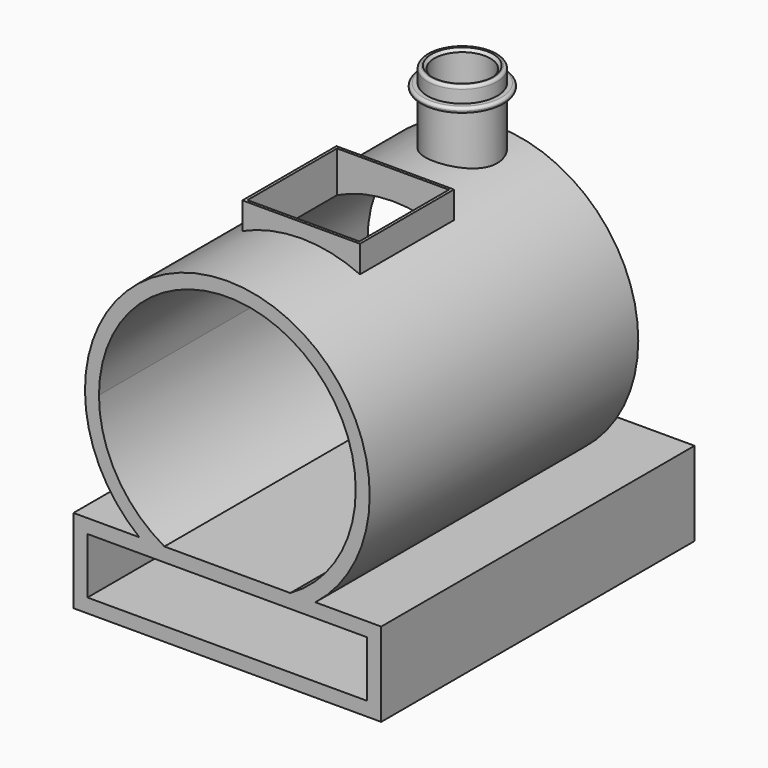
from build123d import *

# Parameters (mm, degrees)
F1_DEPTH      = 120
F0_W          = 5
F0_H          = 5
F2_DEPTH      = 120
F2_DEPTH_BACK = 20
F6_R          = 12.5
F6_R_2        = 10
F7_DEPTH      = 30
F8_R          = 10
F9_DEPTH      = 25
F8_W          = 42
F8_H          = 42
F8_W_2        = 40
F8_H_2        = 40
F10_DEPTH     = 10
F11_DEPTH     = 25
F12_W         = 40
F12_H         = 30
F12_R         = 2.4384
F13_DEPTH     = 25
F16_R         = 15
F16_R_2       = 10
F17_DEPTH     = 2
F18_R         = 0.99999
F19_SIZE      = 1


# Not quite as in the source:
# - a fillet or chamfer is up to 0.001 mm smaller than in the source, because OpenCascade refuses the exact size
# - a feature of the source that left no trace in its solid (it failed there, or was rolled back) is left out
# - a feature names something its author has since deleted; it is built from what else it names


with BuildPart() as f1:
    # F0 (on Front) → F1 (new body)
    with BuildSketch(Plane.XZ):
        with BuildLine():
            ThreePointArc((-22.5, -40), (-39.6160493738, -23.1693468188), (-45.8938993767, 0))
            Line((-45.8938993767, 0), (-50.8938993767, 0))
            ThreePointArc((-50.8938993767, 0), (-45.7803505669, -22.233949171), (-31.4672686099, -40))
            Line((-31.4672686099, -40), (-22.5, -40))
        make_face()
        with BuildLine():
            Line((50.8938993767, 0), (45.8938993767, 0))
            ThreePointArc((45.8938993767, 0), (39.6160493738, -23.1693468188), (22.5, -40))
            Line((22.5, -40), (31.4672686099, -40))
            ThreePointArc((31.4672686099, -40), (45.7803505669, -22.233949171), (50.8938993767, 0))
        make_face()
        with BuildLine():
            ThreePointArc((-45.8938993767, 0), (0, 45.8938993767), (45.8938993767, 0))
            Line((45.8938993767, 0), (50.8938993767, 0))
            ThreePointArc((50.8938993767, 0), (0, 50.8938993767), (-50.8938993767, 0))
            Line((-50.8938993767, 0), (-45.8938993767, 0))
        make_face()
    extrude(amount=F1_DEPTH)

    # F0 (on Front) → F2 (join, two sides)
    with BuildSketch(Plane.XZ) as f2_sk:
        with BuildLine():
            Line((31.4672686099, -40), (22.5, -40))
            ThreePointArc((22.5, -40), (15.954031767, -43.0316031583), (9.0138781887, -45))
            Line((9.0138781887, -45), (23.7737038294, -45))
            ThreePointArc((23.7737038294, -45), (27.7333960958, -42.6737358894), (31.4672686099, -40))
        make_face()
        with BuildLine():
            ThreePointArc((9.0138781887, -45), (15.954031767, -43.0316031583), (22.5, -40))
            Line((22.5, -40), (0, -40))
            Line((0, -40), (-22.5, -40))
            ThreePointArc((-22.5, -40), (-15.954031767, -43.0316031583), (-9.0138781887, -45))
            Line((-9.0138781887, -45), (9.0138781887, -45))
        make_face()
        with BuildLine():
            ThreePointArc((-9.0138781887, -45), (-15.954031767, -43.0316031583), (-22.5, -40))
            Line((-22.5, -40), (-31.4672686099, -40))
            ThreePointArc((-31.4672686099, -40), (-27.7333960958, -42.6737358894), (-23.7737038294, -45))
            Line((-23.7737038294, -45), (-9.0138781887, -45))
        make_face()
        with BuildLine():
            ThreePointArc((-23.7737038294, -45), (-27.7333960958, -42.6737358894), (-31.4672686099, -40))
            Line((-31.4672686099, -40), (-55, -40))
            Line((-55, -40), (-55, -65))
            Line((-55, -65), (-50, -65))
            Line((-50, -65), (-50, -45))
            Line((-50, -45), (-23.7737038294, -45))
        make_face()
        with Locations((-52.5, -67.5)):
            Rectangle(F0_W, F0_H)
        with BuildLine():
            Line((55, -40), (31.4672686099, -40))
            ThreePointArc((31.4672686099, -40), (27.7333960958, -42.6737358894), (23.7737038294, -45))
            Line((23.7737038294, -45), (50, -45))
            Line((50, -45), (50, -65))
            Line((50, -65), (-50, -65))
            Line((-50, -65), (-50, -70))
            Line((-50, -70), (55, -70))
            Line((55, -70), (55, -40))
        make_face()
    extrude(amount=F2_DEPTH)
    extrude(f2_sk.sketch, amount=-F2_DEPTH_BACK)

    # F6 (on offset) → F7 (join)
    with BuildSketch(Plane.XY.offset(76)):
        with Locations((0, -15)):
            Circle(F6_R)
        with Locations((0, -15)):
            Circle(F6_R_2, mode=Mode.SUBTRACT)
    extrude(amount=-F7_DEPTH)

    # F8 (on offset) → F9 (cut)
    with BuildSketch(Plane.XY.offset(56)):
        with Locations((0, -15)):
            Circle(F8_R)
    extrude(amount=-F9_DEPTH, mode=Mode.SUBTRACT)

    # F8 (on offset) → F10 (join)
    with BuildSketch(Plane.XY.offset(56)):
        with Locations((0, -66)):
            Rectangle(F8_W, F8_H)
        with Locations((0, -66)):
            Rectangle(F8_W_2, F8_H_2, mode=Mode.SUBTRACT)
    extrude(amount=-F10_DEPTH)

    # F8 (on offset) → F11 (cut)
    with BuildSketch(Plane.XY.offset(56)):
        with Locations((0, -66)):
            Rectangle(F8_W_2, F8_H_2)
    extrude(amount=-F11_DEPTH, mode=Mode.SUBTRACT)

    # F12 (on face) → F13 (cut)
    with BuildSketch(Plane.XY.offset(-40)):
        with Locations((3.8294e-06, 35)):
            Rectangle(F12_W, F12_H)
        with Locations((0, 60)):
            Circle(F12_R)
    extrude(amount=-F13_DEPTH, mode=Mode.SUBTRACT)

    # F16 (on offset) → F17 (join)
    with BuildSketch(Plane.XY.offset(68.5)):
        with Locations((0, -15)):
            Circle(F16_R)
        with Locations((0, -15)):
            Circle(F16_R_2, mode=Mode.SUBTRACT)
    extrude(amount=F17_DEPTH)

    # F18 (radius 1 in the source; OpenCascade refuses exactly that, so slightly less here)
    f18_edges = [f1.edges().sort_by_distance(p)[0] for p in [
        (-15, -15, 70.5),
        (-15, -15, 68.5),
        (-12.5, -15, 76),
    ]]
    fillet(f18_edges, radius=F18_R)

    # F19
    f19_edges = [f1.edges().sort_by_distance(p)[0] for p in [
        (-10, -15, 76),
    ]]
    chamfer(f19_edges, length=F19_SIZE)


solid = f1.part
